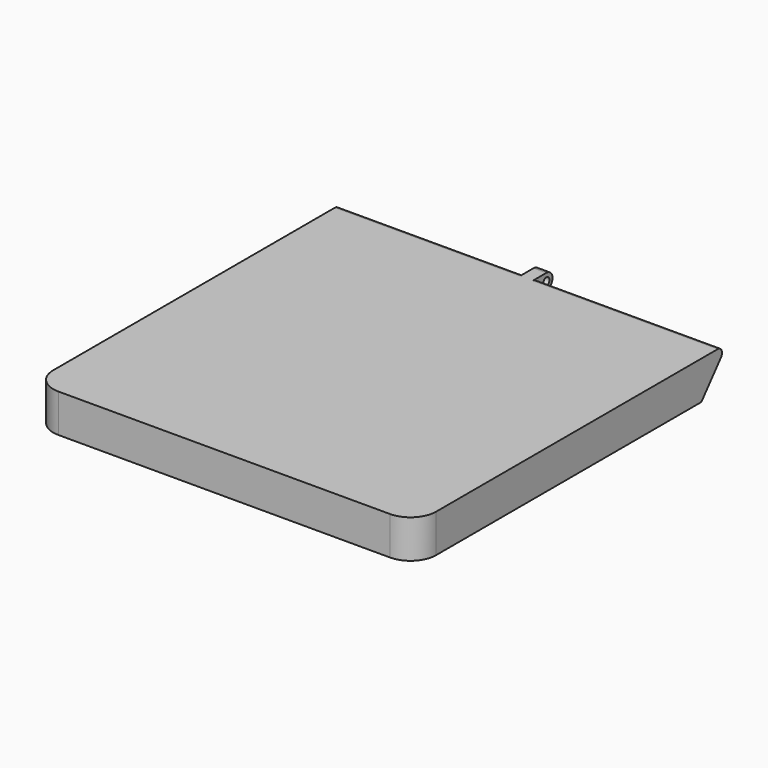
from build123d import *

# Parameters (mm, degrees)
F0_W     = 150
F0_H     = 15
F1_DEPTH = 75
F2_SIZE2 = 10.0691955741
F2_SIZE  = 12
F3_R     = 2
F4_R     = 2.5
F5_DEPTH = 2.5
F6_R     = 1.5
F7_DEPTH = 2.5
F8_R     = 10


with BuildPart() as f1:
    # F0 (on Right) → F1 (new body, symmetric)
    with BuildSketch(Plane.YZ):
        with Locations((15, 24.5)):
            Rectangle(F0_W, F0_H)
    extrude(amount=F1_DEPTH, both=True)

    # F2
    f2_edges = [f1.edges().sort_by_distance(p)[0] for p in [
        (0, 90, 17),
    ]]
    f2_side = f1.faces().sort_by_distance((0, 90, 24.5))[0]
    chamfer(f2_edges, length=F2_SIZE, length2=F2_SIZE2, reference=f2_side)

    # F3
    f3_edges = [f1.edges().sort_by_distance(p)[0] for p in [
        (0, 90, 32),
        (0, 90, 29),
    ]]
    fillet(f3_edges, radius=F3_R)

    # F4 (on Right) → F5 (join, symmetric)
    with BuildSketch(Plane.YZ):
        with BuildLine():
            Line((79.9308044259, 17), (-60, 17))
            Line((-60, 17), (-17.0128849215, -3.2016815445))
            ThreePointArc((-17.0128849215, -3.2016815445), (-2.4781851934, -6.9231586695), (12.4051748829, -5.0277745355))
            Line((12.4051748829, -5.0277745355), (79.9308044259, 17))
        make_face()
        Circle(F4_R, mode=Mode.SUBTRACT)
    extrude(amount=F5_DEPTH, both=True)

    # F6 (on Right) → F7 (join, symmetric)
    with BuildSketch(Plane.YZ):
        with BuildLine():
            Line((94.6649461985, 32), (84.0871334076, 32))
            Line((84.0871334076, 32), (84.0871334076, 26))
            Line((84.0871334076, 26), (94.6649461985, 26))
            ThreePointArc((94.6649461985, 26), (97.6649461985, 29), (94.6649461985, 32))
        make_face()
        with Locations((94.6649461985, 29)):
            Circle(F6_R, mode=Mode.SUBTRACT)
    extrude(amount=F7_DEPTH, both=True)

    # F8
    f8_edges = [f1.edges().sort_by_distance(p)[0] for p in [
        (75, -60, 24.5),
        (-75, -60, 24.5),
    ]]
    fillet(f8_edges, radius=F8_R)


solid = f1.part
